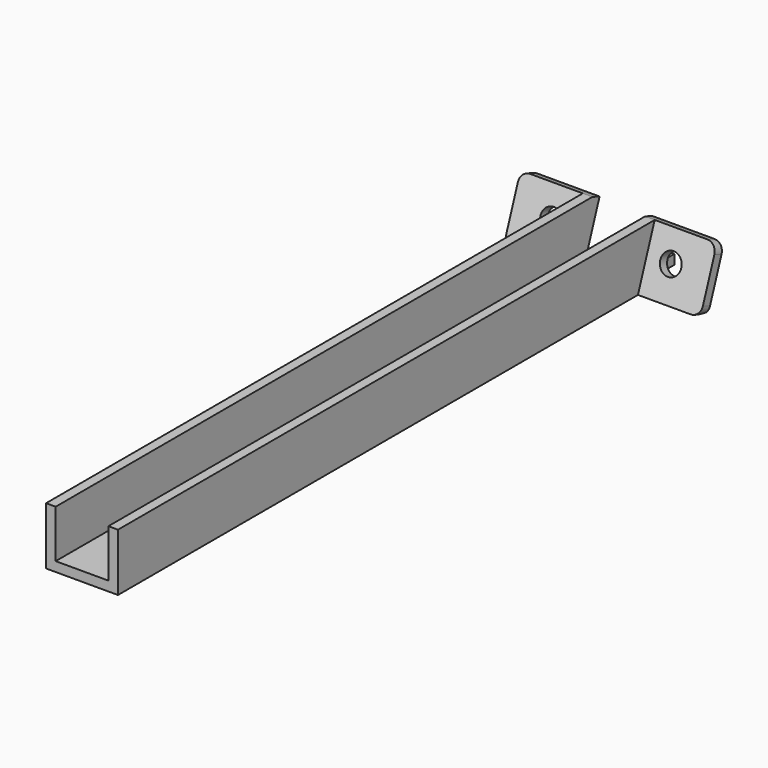
from build123d import *

# Parameters (mm, degrees)
F1_DEPTH  = 140
F3_DEPTH  = 25
F4_W      = 14.9999646693
F4_H      = 12.7701332697
F4_W_2    = 15
F5_DEPTH  = 2
F6_R      = 2
F7_W      = 11
F7_H      = 12
F8_DEPTH  = 2
F10_DEPTH = 50
F12_D     = 4.4


with BuildPart() as f1:
    # F0 (on Front) → F1 (new body)
    with BuildSketch(Plane.XZ):
        Polygon((-5.5, 12), (-7.5, 12), (-7.5, 0), (7.5, 0), (7.5, 12), (5.5, 12), (5.5, 2), (-5.5, 2), align=None)
    extrude(amount=F1_DEPTH)

    # F2 (on face) → F3 (cut)
    with BuildSketch(Plane(origin=(-7.5, 0, 0), x_dir=(0, -1, 0), z_dir=(-1, 0, 0))):
        Polygon((4.3676428112, 0), (0, 12), (0, 0), align=None)
    extrude(amount=-F3_DEPTH, mode=Mode.SUBTRACT)

    # F4 (on face) → F5 (join)
    with BuildSketch(Plane(origin=(0, -3.8567256581, 1.4037333413), x_dir=(-1, 0, 0), z_dir=(0, 0.9396926208, -0.3420201433))):
        with Locations((-12.9999823347, 4.8912448146)):
            Rectangle(F4_W, F4_H)
        with Locations((13, 4.8912448146)):
            Rectangle(F4_W_2, F4_H)
    extrude(amount=F5_DEPTH)

    # F6
    f6_edges = [f1.edges().sort_by_distance(p)[0] for p in [
        (20.499965, 0.939693, 11.65798),
        (-20.5, 0.939693, 11.65798),
        (20.499965, -3.42795, -0.34202),
        (-20.5, -3.42795, -0.34202),
    ]]
    fillet(f6_edges, radius=F6_R)

    # F7 (on face) → F8 (join)
    with BuildSketch(Plane(origin=(0, 0, 0), x_dir=(1, 0, 0), z_dir=(0, 0, -1))):
        with Locations((0, -1.6323571888)):
            Rectangle(F7_W, F7_H)
    extrude(amount=-F8_DEPTH)

    # F9 (on face) → F10 (cut, symmetric)
    with BuildSketch(Plane(origin=(-5.5, 0, 0), x_dir=(0, -1, 0), z_dir=(-1, 0, 0))):
        Polygon((2.2392872662, 0), (-7.6323571888, 0), (-7.6323571888, -1.849311986), (7.0655047894, -1.849311986), (7.0655047894, 0), align=None)
    extrude(amount=F10_DEPTH, both=True, mode=Mode.SUBTRACT)

    # F12 (through all)
    with Locations(Plane(origin=(0, -1.9773404165, 0.7196930546), x_dir=(-1, 0, 0), z_dir=(0, 0.9396926208, -0.3420201433))):
        with Locations((-12.5, 5.2763114494), (12.5, 5.2763114494)):
            Hole(F12_D / 2)


solid = f1.part
